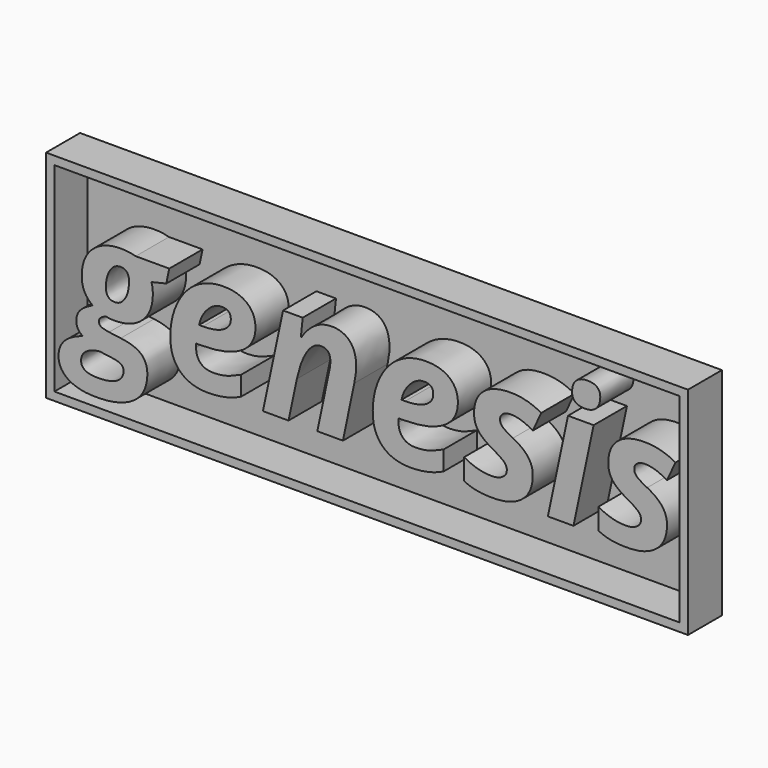
from build123d import *

# Parameters (mm, degrees)
F0_TEXT_SIZE = 106.4066619923
F1_DEPTH     = 25.4
F2_DEPTH     = 25.4
F3_W         = 391.8047249317
F3_H         = 131.831549108
F4_DEPTH     = 0.508
F5_W         = 5.08
F5_H         = 5.08
F5_H_2       = 121.671549108
F5_W_2       = 381.6447249317
F6_DEPTH     = 25.4


# Not quite as in the source:
# - Text() gives the source's letters only with a copy of the font that has no kerning and outlines rounded to 1/6400 em; it was checked with that copy


with BuildPart() as f1:
    # F0 (on Front) → F1 (new body)
    with BuildSketch(Plane.XZ):
        with Locations((-60.2125041187, -31.9805704057)):
            Text('genesis', F0_TEXT_SIZE, font='Open Sans', font_style=FontStyle.BOLDITALIC, text_align=(TextAlign.LEFT, TextAlign.BOTTOM))
    extrude(amount=F1_DEPTH)


with BuildPart() as f2:
    # F0 (on Front) → F2 (new body)
    with BuildSketch(Plane.XZ):
        with Locations((-60.2125041187, -31.9805704057)):
            Text('genesis', F0_TEXT_SIZE, font='Open Sans', font_style=FontStyle.BOLDITALIC, text_align=(TextAlign.LEFT, TextAlign.BOTTOM))
    extrude(amount=F2_DEPTH)


with BuildPart() as f4:
    # F3 (on face) → F4 (new body)
    with BuildSketch(Plane(origin=(0, 0, 0), x_dir=(-1, 0, 0), z_dir=(0, 1, 0))):
        with Locations((-122.114405036, -2.0126961172)):
            Rectangle(F3_W, F3_H)
    extrude(amount=F4_DEPTH)

    # F5 (on face) → F6 (join)
    with BuildSketch(Plane.XZ):
        with Locations((-71.2479574299, 61.3630784369)):
            Rectangle(F5_W, F5_H)
        Polygon((318.0167675018, 63.9030784369), (-68.7079574299, 63.9030784369), (-68.7079574299, 58.8230784369), (312.9367675018, 58.8230784369), (318.0167675018, 58.8230784369), align=None)
        with Locations((-71.2479574299, -2.0126961172)):
            Rectangle(F5_W, F5_H_2)
        with Locations((-71.2479574299, -65.3884706712)):
            Rectangle(F5_W, F5_H)
        with Locations((315.4767675018, -2.0126961172)):
            Rectangle(F5_W, F5_H_2)
        with Locations((122.114405036, -65.3884706712)):
            Rectangle(F5_W_2, F5_H)
        with Locations((315.4767675018, -65.3884706712)):
            Rectangle(F5_W, F5_H)
    extrude(amount=F6_DEPTH)


solid = Compound([f1.part, f2.part, f4.part])
